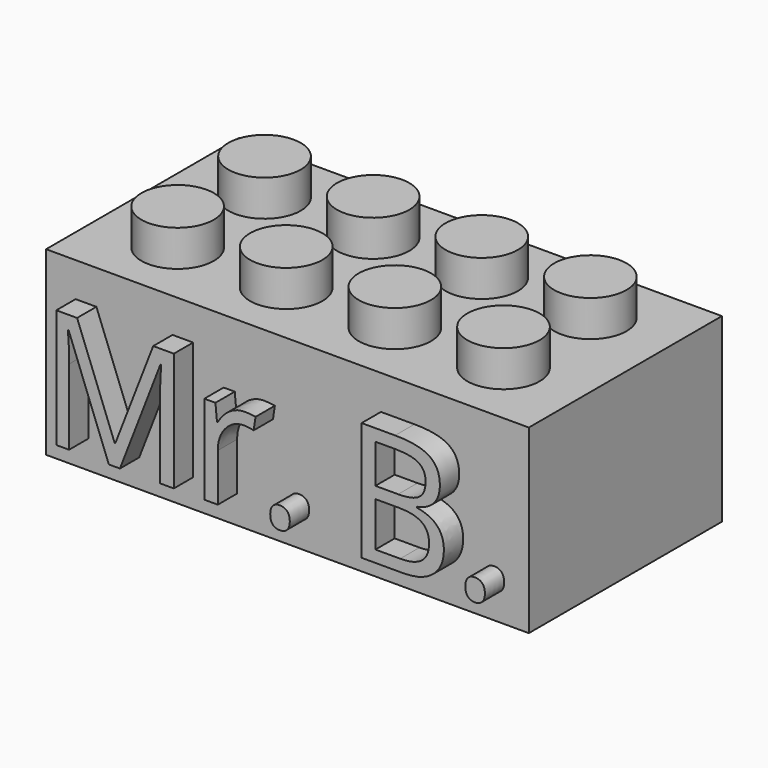
from build123d import *

# Parameters (mm, degrees)
F0_R         = 3
F1_DEPTH     = 18
F0_W         = 40
F0_H         = 20
F2_DEPTH     = 15
F3_TEXT_SIZE = 13.7707179723
F4_DEPTH     = 2


# Not quite as in the source:
# - Text() gives the source's letters only with a copy of the font that has no kerning and outlines rounded to 1/6400 em; it was checked with that copy


with BuildPart() as f1:
    # F0 (on Top) → F1 (new body)
    with BuildSketch(Plane.XY):
        with Locations((-7.7492720579, 1.4983603805)):
            Circle(F0_R)
    extrude(amount=F1_DEPTH)


with BuildPart() as f1b:
    # F0 (on Top) → F1, piece 2 (new body)
    with BuildSketch(Plane.XY):
        with Locations((1.2507279421, -7.5016396195)):
            Circle(F0_R)
    extrude(amount=F1_DEPTH)


with BuildPart() as f1c:
    # F0 (on Top) → F1, piece 3 (new body)
    with BuildSketch(Plane.XY):
        with Locations((1.2507279421, 1.4983603805)):
            Circle(F0_R)
    extrude(amount=F1_DEPTH)


with BuildPart() as f1d:
    # F0 (on Top) → F1, piece 4 (new body)
    with BuildSketch(Plane.XY):
        with Locations((10.2507279421, -7.5016396195)):
            Circle(F0_R)
    extrude(amount=F1_DEPTH)


with BuildPart() as f1e:
    # F0 (on Top) → F1, piece 5 (new body)
    with BuildSketch(Plane.XY):
        with Locations((10.2507279421, 1.4983603805)):
            Circle(F0_R)
    extrude(amount=F1_DEPTH)


with BuildPart() as f1f:
    # F0 (on Top) → F1, piece 6 (new body)
    with BuildSketch(Plane.XY):
        with Locations((19.2507279421, -7.5016396195)):
            Circle(F0_R)
    extrude(amount=F1_DEPTH)


with BuildPart() as f1g:
    # F0 (on Top) → F1, piece 7 (new body)
    with BuildSketch(Plane.XY):
        with Locations((19.2507279421, 1.4983603805)):
            Circle(F0_R)
    extrude(amount=F1_DEPTH)


with BuildPart() as f1h:
    # F0 (on Top) → F1, piece 8 (new body)
    with BuildSketch(Plane.XY):
        with Locations((-7.7492720579, -7.5016396195)):
            Circle(F0_R)
    extrude(amount=F1_DEPTH)


with BuildPart() as f2:
    # F0 (on Top) → F2 (new body)
    with BuildSketch(Plane.XY):
        with Locations((5.7507279421, -3.0016396195)):
            Rectangle(F0_W, F0_H)
        with Locations((-7.7492720579, -7.5016396195)):
            Circle(F0_R, mode=Mode.SUBTRACT)
        with Locations((1.2507279421, -7.5016396195)):
            Circle(F0_R, mode=Mode.SUBTRACT)
        with Locations((10.2507279421, -7.5016396195)):
            Circle(F0_R, mode=Mode.SUBTRACT)
        with Locations((19.2507279421, -7.5016396195)):
            Circle(F0_R, mode=Mode.SUBTRACT)
        with Locations((-7.7492720579, 1.4983603805)):
            Circle(F0_R, mode=Mode.SUBTRACT)
        with Locations((1.2507279421, 1.4983603805)):
            Circle(F0_R, mode=Mode.SUBTRACT)
        with Locations((10.2507279421, 1.4983603805)):
            Circle(F0_R, mode=Mode.SUBTRACT)
        with Locations((19.2507279421, 1.4983603805)):
            Circle(F0_R, mode=Mode.SUBTRACT)
    extrude(amount=F2_DEPTH)

    # F3 (on face) → F4 (join)
    with BuildSketch(Plane.XZ.offset(13.0016396195)):
        with Locations((-13.1525602192, 2.3234861437)):
            Text('Mr. B.', F3_TEXT_SIZE, font='Open Sans', text_align=(TextAlign.LEFT, TextAlign.BOTTOM))
    extrude(amount=F4_DEPTH)


solid = Compound([f1.part, f1b.part, f1c.part, f1d.part, f1e.part, f1f.part, f1g.part, f1h.part, f2.part])
